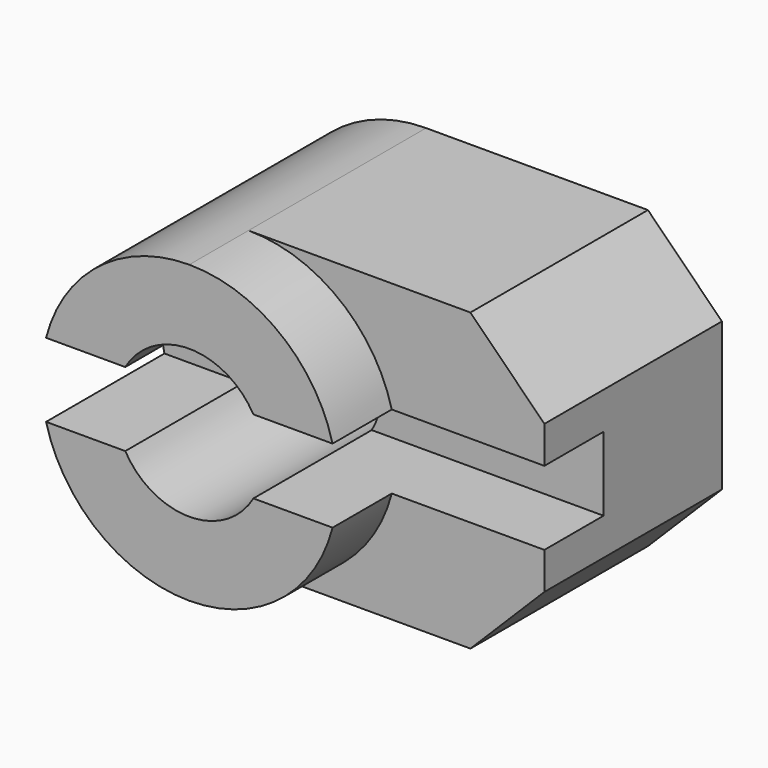
from build123d import *

# Parameters (mm, degrees)
F1_DEPTH = 10
F2_DEPTH = 10
F3_DEPTH = 5


# Not quite as in the source:
# - after a boolean that leaves OpenCascade's solid faulty, fix() repairs it


with BuildPart() as f1:
    # F0 (on Front) → F1 (new body)
    with BuildSketch(Plane.XZ):
        with BuildLine():
            Line((4.3301270189, 2.5), (9.6824583655, 2.5))
            ThreePointArc((9.6824583655, 2.5), (6.123724357, 7.9056941504), (0, 10))
            ThreePointArc((0, 10), (-6.123724357, 7.9056941504), (-9.6824583655, 2.5))
            Line((-9.6824583655, 2.5), (-4.3301270189, 2.5))
            ThreePointArc((-4.3301270189, 2.5), (0, 5), (4.3301270189, 2.5))
        make_face()
        with BuildLine():
            Line((-4.3301270189, -2.5), (-9.6824583655, -2.5))
            ThreePointArc((-9.6824583655, -2.5), (-6.123724357, -7.9056941504), (0, -10))
            ThreePointArc((0, -10), (6.123724357, -7.9056941504), (9.6824583655, -2.5))
            Line((9.6824583655, -2.5), (4.3301270189, -2.5))
            ThreePointArc((4.3301270189, -2.5), (0, -5), (-4.3301270189, -2.5))
        make_face()
    extrude(amount=F1_DEPTH)

    # F0 (on Front) → F2 (join)
    with BuildSketch(Plane.XZ):
        with BuildLine():
            ThreePointArc((0, 10), (6.123724357, 7.9056941504), (9.6824583655, 2.5))
            Line((9.6824583655, 2.5), (20, 2.5))
            Line((20, 2.5), (20, 5))
            Line((20, 5), (15, 10))
            Line((15, 10), (0, 10))
        make_face()
        with BuildLine():
            Line((20, -5), (20, -2.5))
            Line((20, -2.5), (9.6824583655, -2.5))
            ThreePointArc((9.6824583655, -2.5), (6.123724357, -7.9056941504), (0, -10))
            Line((0, -10), (15, -10))
            Line((15, -10), (20, -5))
        make_face()
        with BuildLine():
            Line((20, 2.5), (9.6824583655, 2.5))
            Line((9.6824583655, 2.5), (4.3301270189, 2.5))
            ThreePointArc((4.3301270189, 2.5), (4.8296291314, 1.2940952255), (5, 0))
            ThreePointArc((5, 0), (4.8296291314, -1.2940952255), (4.3301270189, -2.5))
            Line((4.3301270189, -2.5), (9.6824583655, -2.5))
            Line((9.6824583655, -2.5), (20, -2.5))
            Line((20, -2.5), (20, 2.5))
        make_face()
        with BuildLine():
            Line((4.3301270189, 2.5), (9.6824583655, 2.5))
            ThreePointArc((9.6824583655, 2.5), (6.123724357, 7.9056941504), (0, 10))
            ThreePointArc((0, 10), (-6.123724357, 7.9056941504), (-9.6824583655, 2.5))
            Line((-9.6824583655, 2.5), (-4.3301270189, 2.5))
            ThreePointArc((-4.3301270189, 2.5), (0, 5), (4.3301270189, 2.5))
        make_face()
        with BuildLine():
            Line((-4.3301270189, 2.5), (-9.6824583655, 2.5))
            ThreePointArc((-9.6824583655, 2.5), (-10, 0), (-9.6824583655, -2.5))
            Line((-9.6824583655, -2.5), (-4.3301270189, -2.5))
            ThreePointArc((-4.3301270189, -2.5), (-5, 0), (-4.3301270189, 2.5))
        make_face()
        with BuildLine():
            Line((-4.3301270189, -2.5), (-9.6824583655, -2.5))
            ThreePointArc((-9.6824583655, -2.5), (-6.123724357, -7.9056941504), (0, -10))
            ThreePointArc((0, -10), (6.123724357, -7.9056941504), (9.6824583655, -2.5))
            Line((9.6824583655, -2.5), (4.3301270189, -2.5))
            ThreePointArc((4.3301270189, -2.5), (0, -5), (-4.3301270189, -2.5))
        make_face()
    extrude(amount=-F2_DEPTH)

    add(f1.part.fix(), mode=Mode.REPLACE)

    # F0 (on Front) → F3 (join)
    with BuildSketch(Plane.XZ):
        with BuildLine():
            ThreePointArc((0, 10), (6.123724357, 7.9056941504), (9.6824583655, 2.5))
            Line((9.6824583655, 2.5), (20, 2.5))
            Line((20, 2.5), (20, 5))
            Line((20, 5), (15, 10))
            Line((15, 10), (0, 10))
        make_face()
        with BuildLine():
            Line((20, -5), (20, -2.5))
            Line((20, -2.5), (9.6824583655, -2.5))
            ThreePointArc((9.6824583655, -2.5), (6.123724357, -7.9056941504), (0, -10))
            Line((0, -10), (15, -10))
            Line((15, -10), (20, -5))
        make_face()
    extrude(amount=F3_DEPTH)


solid = f1.part
